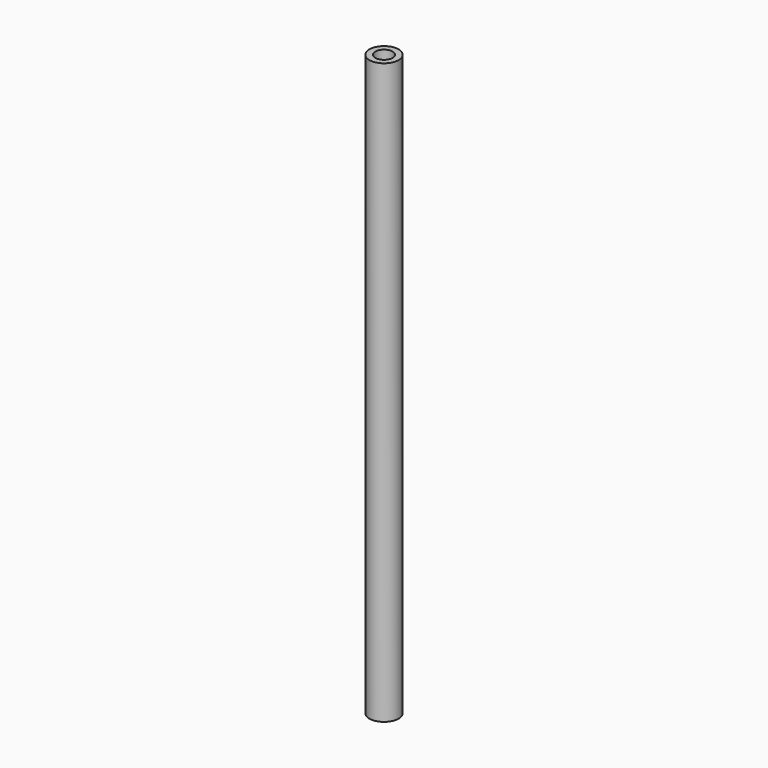
from build123d import *

# Parameters (mm, degrees)
F1_R     = 10.715625
F1_R_2   = 6.35
F2_DEPTH = 425.45


# Not quite as in the source:
# - a variable given as a bare number and used for a length is read in inches; the dataset says mm whatever the document's units were


with BuildPart() as f2:
    # F1 (on Top) → F2 (new body)
    with BuildSketch(Plane.XY):
        Circle(F1_R)
        Circle(F1_R_2, mode=Mode.SUBTRACT)
    extrude(amount=F2_DEPTH)


solid = f2.part
